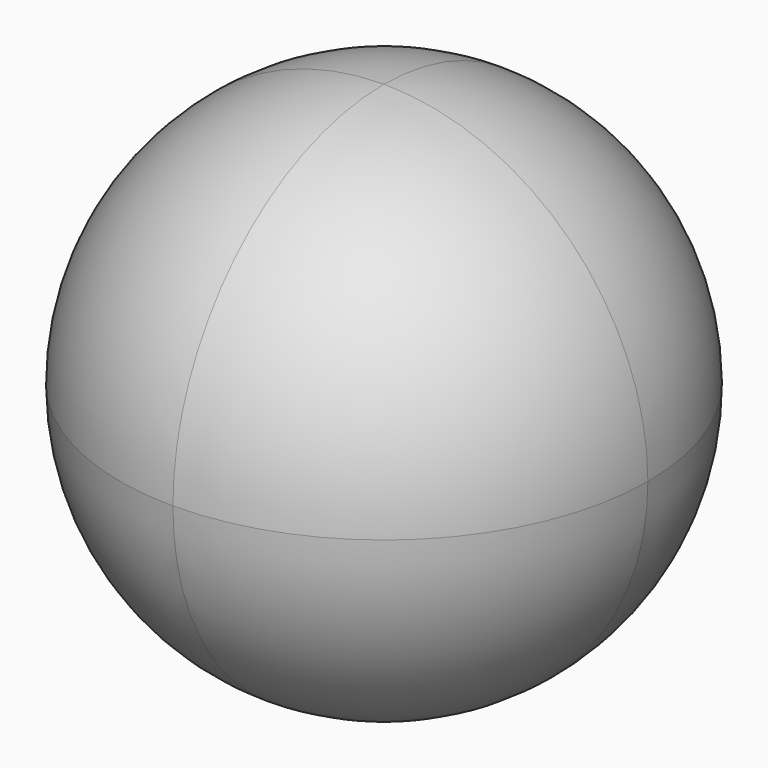
from build123d import *

# Parameters (mm, degrees)
F0_W     = 40
F0_H     = 40
F1_DEPTH = 40
F2_R     = 19.99999


# Not quite as in the source:
# - a fillet or chamfer is up to 0.001 mm smaller than in the source, because OpenCascade refuses the exact size


with BuildPart() as f1:
    # F0 (on Top) → F1 (new body)
    with BuildSketch(Plane.XY):
        with Locations((-28.959679883, 29.835797905)):
            Rectangle(F0_W, F0_H)
    extrude(amount=F1_DEPTH)

    # F2 (radius 20 in the source; OpenCascade refuses exactly that, so slightly less here)
    f2_edges = [f1.edges().sort_by_distance(p)[0] for p in [
        (-8.95968, 49.835798, 20),
        (-48.95968, 9.835798, 20),
        (-48.95968, 49.835798, 20),
        (-28.95968, 49.835798, 0),
        (-28.95968, 49.835798, 40),
        (-48.95968, 29.835798, 40),
        (-28.95968, 9.835798, 40),
        (-8.95968, 29.835798, 40),
        (-48.95968, 29.835798, 0),
        (-8.95968, 9.835798, 20),
        (-8.95968, 29.835798, 0),
        (-28.95968, 9.835798, 0),
    ]]
    fillet(f2_edges, radius=F2_R)


solid = f1.part
